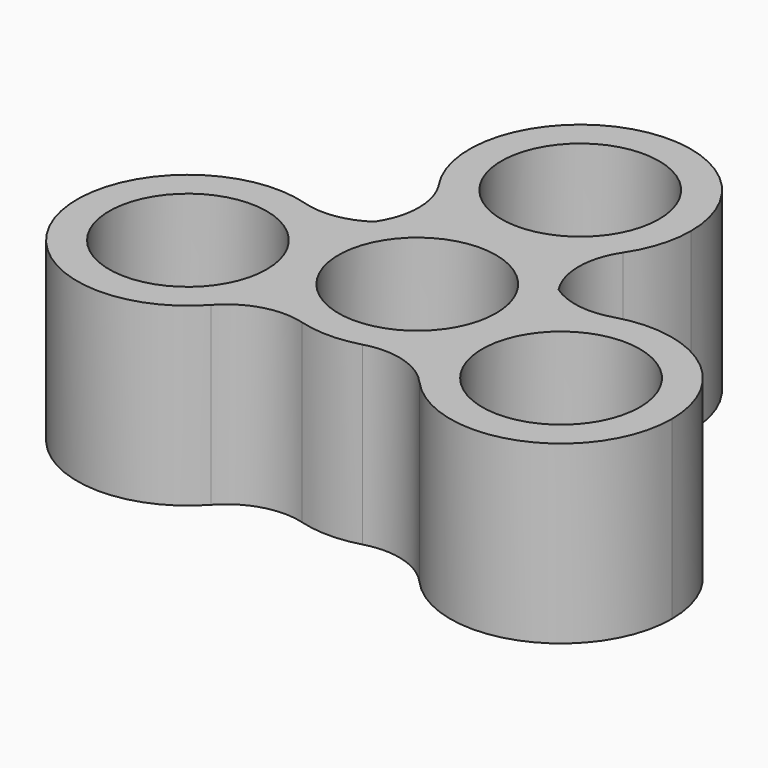
from build123d import *

# Parameters (mm, degrees)
F0_R        = 11.3737467854
F1_DEPTH    = 25.4
F2_R        = 10.5009772193
F3_R        = 10.4902
F4_R        = 10.4902
F5_T1_DEPTH = 25.4
F6_R        = 10.4902
F7_T1_DEPTH = 25.4


# Not quite as in the source:
# - a fillet or chamfer that OpenCascade refuses, or shapes differently, is made with other operations: its cross-section is extruded or revolved along the edge and cut away or added


with BuildPart() as f1:
    # F0 (on Top) → F1 (new body)
    with BuildSketch(Plane.XY):
        with BuildLine():
            ThreePointArc((6.2894283282, 14.6999955177), (13.345564471, 20.5941585441), (15.9889579684, 29.3999910355))
            ThreePointArc((15.9889579684, 29.3999910355), (-8.8058324914, 42.7455555065), (-6.2894283282, 14.6999955177))
            ThreePointArc((-6.2894283282, 14.6999955177), (0, 15.9889579684), (6.2894283282, 14.6999955177))
        make_face()
        with Locations((0, 29.3999910355)):
            Circle(F0_R, mode=Mode.SUBTRACT)
        with BuildLine():
            ThreePointArc((6.2894283282, 14.6999955177), (0, 13.411033067), (-6.2894283282, 14.6999955177))
            ThreePointArc((-6.2894283282, 14.6999955177), (-12.2780666284, 10.2418678368), (-15.5897168926, 3.5507047362))
            ThreePointArc((-15.5897168926, 3.5507047362), (-12.1065325646, -1.6446399909), (-10.8830575897, -7.7787486371))
            ThreePointArc((-10.8830575897, -7.7787486371), (-10.983181349, -9.5652884184), (-11.2822986655, -11.3294533733))
            ThreePointArc((-11.2822986655, -11.3294533733), (0.0583928669, -15.9888513405), (11.3647491723, -11.246744114))
            ThreePointArc((11.3647491723, -11.246744114), (11.6102118149, -3.3482637899), (15.6083251298, 3.467991286))
            ThreePointArc((15.6083251298, 3.467991286), (12.3051770158, 10.209279873), (6.2894283282, 14.6999955177))
        make_face()
        Circle(F0_R, mode=Mode.SUBTRACT)
        with BuildLine():
            ThreePointArc((42.9620322705, -7.778752828), (33.0532173957, 7.0090339191), (15.6083251298, 3.467991286))
            ThreePointArc((15.6083251298, 3.467991286), (15.893514894, 1.7444085615), (15.9889579684, 0))
            ThreePointArc((15.9889579684, 0), (14.7877867471, -6.0801430936), (11.3647491723, -11.246744114))
            ThreePointArc((11.3647491723, -11.246744114), (28.7174828636, -23.6722677221), (42.9620322705, -7.778752828))
        make_face()
        with Locations((26.9730743021, -7.778752828)):
            Circle(F0_R, mode=Mode.SUBTRACT)
        with BuildLine():
            ThreePointArc((-11.2822986655, -11.3294533733), (-15.3584205367, -4.4458627437), (-15.5897168926, 3.5507047362))
            ThreePointArc((-15.5897168926, 3.5507047362), (-42.2304360948, -12.2246113807), (-11.2822986655, -11.3294533733))
        make_face()
        with Locations((-26.8720155582, -7.7787486371)):
            Circle(F0_R, mode=Mode.SUBTRACT)
        with BuildLine():
            ThreePointArc((-10.8830575897, -7.7787486371), (-12.1065325646, -1.6446399909), (-15.5897168926, 3.5507047362))
            ThreePointArc((-15.5897168926, 3.5507047362), (-15.3584205367, -4.4458627437), (-11.2822986655, -11.3294533733))
            ThreePointArc((-11.2822986655, -11.3294533733), (-10.983181349, -9.5652884184), (-10.8830575897, -7.7787486371))
        make_face()
        with BuildLine():
            ThreePointArc((6.2894283282, 14.6999955177), (0, 15.9889579684), (-6.2894283282, 14.6999955177))
            ThreePointArc((-6.2894283282, 14.6999955177), (0, 13.411033067), (6.2894283282, 14.6999955177))
        make_face()
        with BuildLine():
            ThreePointArc((15.9889579684, 0), (15.893514894, 1.7444085615), (15.6083251298, 3.467991286))
            ThreePointArc((15.6083251298, 3.467991286), (11.6102118149, -3.3482637899), (11.3647491723, -11.246744114))
            ThreePointArc((11.3647491723, -11.246744114), (14.7877867471, -6.0801430936), (15.9889579684, 0))
        make_face()
    extrude(amount=F1_DEPTH)

    # F2
    f2_edges = [f1.edges().sort_by_distance(p)[0] for p in [
        (-11.282299, -11.329453, 12.7),
    ]]
    fillet(f2_edges, radius=F2_R)

    # F3
    f3_edges = [f1.edges().sort_by_distance(p)[0] for p in [
        (6.289428, 14.699996, 12.7),
    ]]
    fillet(f3_edges, radius=F3_R)

    # F4
    f4_edges = [f1.edges().sort_by_distance(p)[0] for p in [
        (11.364749, -11.246744, 12.7),
    ]]
    fillet(f4_edges, radius=F4_R)

    # F5: fillet of radius 10.4902 on 1 edges, made by hand

    # F5_s2 → F5_t1 (join)
    with BuildSketch(Plane.XY):
        with BuildLine():
            ThreePointArc((22.2888959377, 7.5086684708), (17.6379410744, 7.1677184148), (13.298783115, 8.8763249477))
            ThreePointArc((13.298783115, 8.8763249477), (14.7043444266, 6.2792540878), (15.6083251298, 3.467991286))
            ThreePointArc((15.6083251298, 3.467991286), (18.6981853725, 5.9023651862), (22.2888959377, 7.5086684708))
        make_face()
    extrude(amount=F5_T1_DEPTH)

    # F6
    f6_edges = [f1.edges().sort_by_distance(p)[0] for p in [
        (-6.289428, 14.699996, 12.7),
    ]]
    fillet(f6_edges, radius=F6_R)

    # F7: fillet of radius 10.4902 on 1 edges, made by hand

    # F7_s2 → F7_t1 (join)
    with BuildSketch(Plane.XY):
        with BuildLine():
            ThreePointArc((-13.298783115, 8.8763249477), (-17.6110780147, 7.1883289802), (-22.2299741232, 7.5215202571))
            ThreePointArc((-22.2299741232, 7.5215202571), (-18.6660423749, 5.9438160297), (-15.5897168926, 3.5507047362))
            ThreePointArc((-15.5897168926, 3.5507047362), (-14.6876450063, 6.3182166063), (-13.298783115, 8.8763249477))
        make_face()
    extrude(amount=F7_T1_DEPTH)


solid = f1.part
